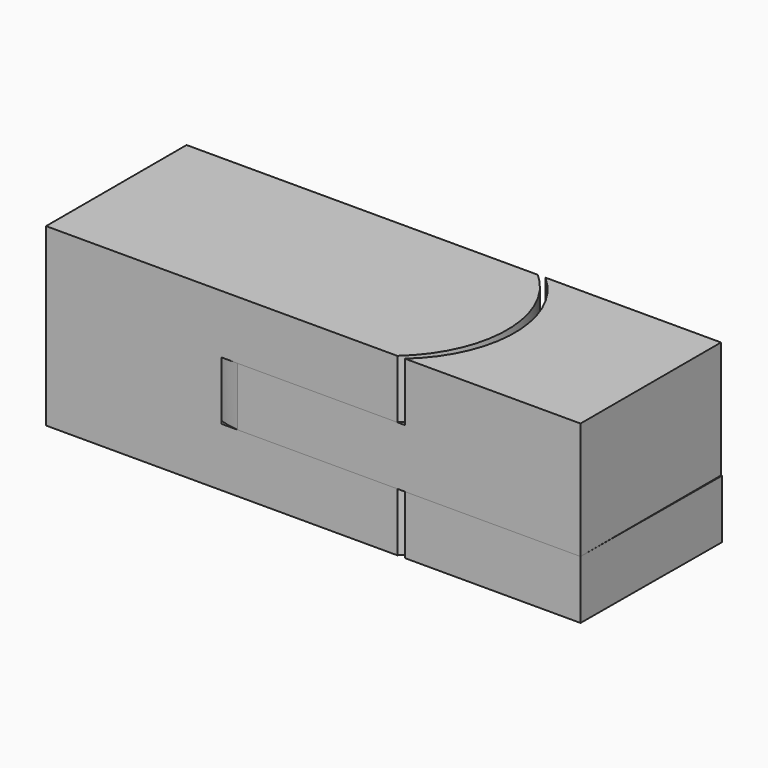
from build123d import *

# Parameters (mm, degrees)
F1_DEPTH = 5
F2_R     = 4
F3_DEPTH = 5
F2_R_2   = 4.1526486357
F4_DEPTH = 5
F6_DEPTH = 5
F7_DEPTH = 5


with BuildPart() as f1:
    # F0 (on Top) → F1 (new body)
    with BuildSketch(Plane.XY):
        with BuildLine():
            Line((15, 7.5), (-15, 7.5))
            Line((-15, 7.5), (-15, -7.5))
            Line((-15, -7.5), (15, -7.5))
            ThreePointArc((15, -7.5), (18.3856217223, 0), (15, 7.5))
        make_face()
    extrude(amount=F1_DEPTH)

    # F2 (on face) → F3 (join)
    with BuildSketch(Plane.XY.offset(5)):
        with BuildLine():
            Line((0, 7.5), (-15, 7.5))
            Line((-15, 7.5), (-15, -7.5))
            Line((-15, -7.5), (0, -7.5))
            ThreePointArc((0, -7.5), (-5.8695986214, 0), (0, 7.5))
        make_face()
        with Locations((7.5, 0)):
            Circle(F2_R)
    extrude(amount=F3_DEPTH)

    # F5 (on face) → F7 (join)
    with BuildSketch(Plane.XY.offset(10)):
        with BuildLine():
            ThreePointArc((15, -7.5), (18.3856217223, 0), (15, 7.5))
            Line((15, 7.5), (0, 7.5))
            ThreePointArc((0, 7.5), (-5.8695986214, 0), (0, -7.5))
            Line((0, -7.5), (15, -7.5))
        make_face()
        with BuildLine():
            ThreePointArc((0, -7.5), (-5.8695986214, 0), (0, 7.5))
            Line((0, 7.5), (-15, 7.5))
            Line((-15, 7.5), (-15, -7.5))
            Line((-15, -7.5), (0, -7.5))
        make_face()
    extrude(amount=F7_DEPTH)


with BuildPart() as f1b:
    # F0 (on Top) → F1, piece 2 (new body)
    with BuildSketch(Plane.XY):
        with BuildLine():
            Line((30.7328099012, 7.5), (15.7328099012, 7.5))
            ThreePointArc((15.7328099012, 7.5), (19.078910202, -0.0177155588), (15.6538608473, -7.4997922335))
            Line((15.6538608473, -7.4997922335), (30.6538608473, -7.4997922335))
            Line((30.6538608473, -7.4997922335), (30.7328099012, 7.5))
        make_face()
    extrude(amount=F1_DEPTH)

    # F2 (on face) → F4 (join)
    with BuildSketch(Plane.XY.offset(5)):
        with BuildLine():
            Line((15, 7.5), (1.3659824617, 7.5))
            ThreePointArc((1.3659824617, 7.5), (-5.5026358727, 0), (1.3659824617, -7.5))
            Line((1.3659824617, -7.5), (15, -7.5))
            ThreePointArc((15, -7.5), (18.3856217223, 0), (15, 7.5))
        make_face()
        with Locations((7.5, 0)):
            Circle(F2_R_2, mode=Mode.SUBTRACT)
        with BuildLine():
            Line((30.6538597538, 7.5), (15, 7.5))
            ThreePointArc((15, 7.5), (18.3856217223, 0), (15, -7.5))
            Line((15, -7.5), (30.6538597538, -7.5))
            Line((30.6538597538, -7.5), (30.6538597538, 7.5))
        make_face()
    extrude(amount=F4_DEPTH)

    # F5 (on face) → F6 (join)
    with BuildSketch(Plane.XY.offset(10)):
        with BuildLine():
            Line((30.6538597538, 7.5), (15.6538597538, 7.5))
            ThreePointArc((15.6538597538, 7.5), (19.0394814761, 0), (15.6538597538, -7.5))
            Line((15.6538597538, -7.5), (30.6538597538, -7.5))
            Line((30.6538597538, -7.5), (30.6538597538, 7.5))
        make_face()
    extrude(amount=F6_DEPTH)


solid = Compound([f1.part, f1b.part])
